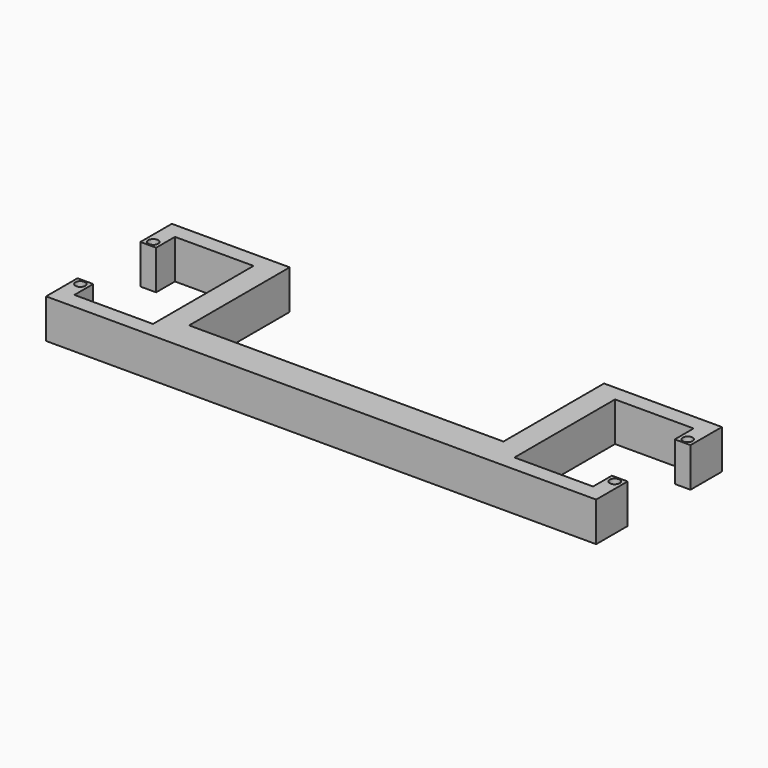
from build123d import *

# Parameters (mm, degrees)
F0_R     = 0.396875
F0_W     = 25.4
F0_H     = 2.54
F1_DEPTH = 3.175


# Not quite as in the source:
# - a feature names something its author has since deleted; it is built from what else it names


with BuildPart() as f1:
    # F0 (on Top) → F1 (new body)
    with BuildSketch(Plane.XY):
        Polygon((-12.7, 11.43), (-22.225, 11.43), (-22.225, 8.255), (-20.955, 8.255), (-20.955, 10.16), (-14.605, 10.16), (-14.605, 0), (-20.955, 0), (-20.955, 1.905), (-22.225, 1.905), (-22.225, -1.27), (-12.7, -1.27), (-12.7, 1.27), align=None)
        with Locations((-21.59, 1.397)):
            Circle(F0_R, mode=Mode.SUBTRACT)
        with Locations((-21.59, 8.763)):
            Circle(F0_R, mode=Mode.SUBTRACT)
        Rectangle(F0_W, F0_H)
        Polygon((12.7, 11.43), (12.7, 1.27), (12.7, -1.27), (22.225, -1.27), (22.225, 1.905), (20.955, 1.905), (20.955, 0), (14.605, 0), (14.605, 10.16), (20.955, 10.16), (20.955, 8.255), (22.225, 8.255), (22.225, 11.43), align=None)
        with Locations((21.59, 1.397)):
            Circle(F0_R, mode=Mode.SUBTRACT)
        with Locations((21.59, 8.763)):
            Circle(F0_R, mode=Mode.SUBTRACT)
    extrude(amount=F1_DEPTH)


solid = f1.part
